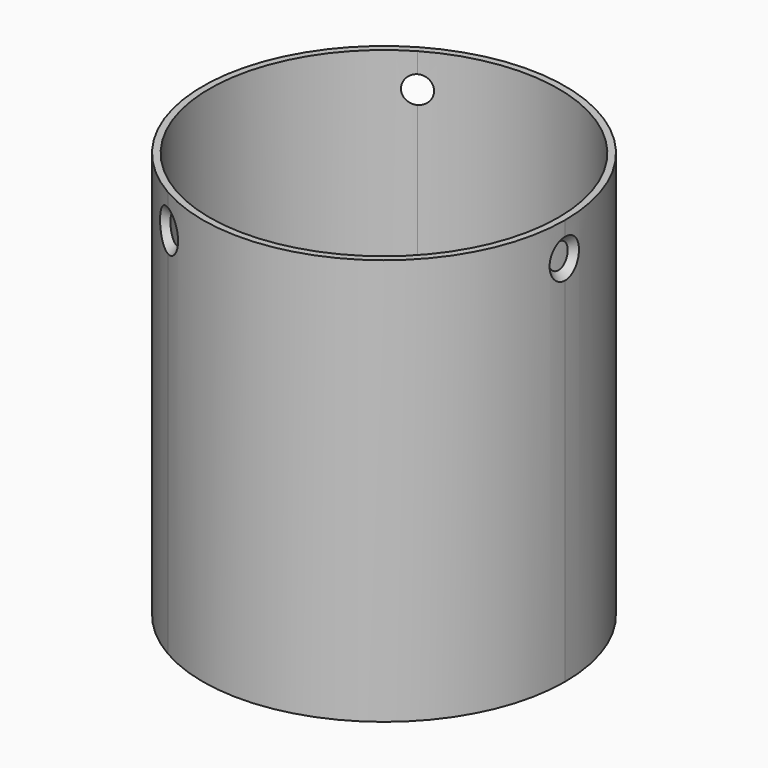
from build123d import *

# Parameters (mm, degrees)
F1_DEPTH             = 60
F2_DEPTH             = 58
F9_D                 = 3.2
F9_DEPTH             = 4
F9_CSINK_D           = 6
F9_CSINK_ANGLE       = 90
F9_TIP               = 0.9613769904
F9_ON_F6_D           = 3.2
F9_ON_F6_DEPTH       = 4
F9_ON_F6_CSINK_D     = 6
F9_ON_F6_CSINK_ANGLE = 90
F9_ON_F6_TIP         = 0.9613769904
F9_ON_F8_D           = 3.2
F9_ON_F8_DEPTH       = 4
F9_ON_F8_CSINK_D     = 6
F9_ON_F8_CSINK_ANGLE = 90
F9_ON_F8_TIP         = 0.9613769904


# Not quite as in the source:
# - a feature names something its author has since deleted; it is built from what else it names


with BuildPart() as f1:
    # F0 (on Top) → F1 (new body)
    with BuildSketch(Plane.XY):
        with BuildLine():
            ThreePointArc((-13.375, -23.1661795512), (13.375, -23.1661795512), (26.75, 0))
            ThreePointArc((26.75, 0), (13.375, 23.1661795512), (-13.375, 23.1661795512))
            Line((-13.375, 23.1661795512), (-12.875, 22.3001541474))
            ThreePointArc((-12.875, 22.3001541474), (12.875, 22.3001541474), (25.75, 0))
            ThreePointArc((25.75, 0), (12.875, -22.3001541474), (-12.875, -22.3001541474))
            Line((-12.875, -22.3001541474), (-13.375, -23.1661795512))
        make_face()
        with BuildLine():
            Line((-12.875, 22.3001541474), (-13.375, 23.1661795512))
            ThreePointArc((-13.375, 23.1661795512), (-26.75, 0), (-13.375, -23.1661795512))
            Line((-13.375, -23.1661795512), (-12.875, -22.3001541474))
            ThreePointArc((-12.875, -22.3001541474), (-25.75, 0), (-12.875, 22.3001541474))
        make_face()
        with BuildLine():
            ThreePointArc((25.75, 0), (12.875, 22.3001541474), (-12.875, 22.3001541474))
            Line((-12.875, 22.3001541474), (0, 0))
            Line((0, 0), (-12.875, -22.3001541474))
            ThreePointArc((-12.875, -22.3001541474), (12.875, -22.3001541474), (25.75, 0))
        make_face()
        with BuildLine():
            Line((0, 0), (-12.875, 22.3001541474))
            ThreePointArc((-12.875, 22.3001541474), (-25.75, 0), (-12.875, -22.3001541474))
            Line((-12.875, -22.3001541474), (0, 0))
        make_face()
    extrude(amount=-F1_DEPTH)

    # F0 (on Top) → F2 (cut)
    with BuildSketch(Plane.XY):
        with BuildLine():
            ThreePointArc((25.75, 0), (12.875, 22.3001541474), (-12.875, 22.3001541474))
            Line((-12.875, 22.3001541474), (0, 0))
            Line((0, 0), (-12.875, -22.3001541474))
            ThreePointArc((-12.875, -22.3001541474), (12.875, -22.3001541474), (25.75, 0))
        make_face()
        with BuildLine():
            Line((0, 0), (-12.875, 22.3001541474))
            ThreePointArc((-12.875, 22.3001541474), (-25.75, 0), (-12.875, -22.3001541474))
            Line((-12.875, -22.3001541474), (0, 0))
        make_face()
    extrude(amount=-F2_DEPTH, mode=Mode.SUBTRACT)

    # F9
    with Locations(Plane(origin=(-13.375, 23.1661795512, 0), x_dir=(-0.8660254038, -0.5, 0), z_dir=(-0.5, 0.8660254038, 0))):
        with Locations((0, -5)):
            CounterSinkHole(F9_D / 2, F9_CSINK_D / 2, depth=F9_DEPTH, counter_sink_angle=F9_CSINK_ANGLE)
            with Locations((0, 0, -(F9_DEPTH + F9_TIP / 2))):  # 118° drill point
                Cone(0, F9_D / 2, F9_TIP, mode=Mode.SUBTRACT)

    # F9 on F6
    with Locations(Plane.YZ.offset(26.9)):
        with Locations((0, -5)):
            CounterSinkHole(F9_ON_F6_D / 2, F9_ON_F6_CSINK_D / 2, depth=F9_ON_F6_DEPTH, counter_sink_angle=F9_ON_F6_CSINK_ANGLE)
            with Locations((0, 0, -(F9_ON_F6_DEPTH + F9_ON_F6_TIP / 2))):  # 118° drill point
                Cone(0, F9_ON_F6_D / 2, F9_ON_F6_TIP, mode=Mode.SUBTRACT)

    # F9 on F8
    with Locations(Plane(origin=(-13.375, -23.1661795512, 0), x_dir=(0.8660254038, -0.5, 0), z_dir=(-0.5, -0.8660254038, 0))):
        with Locations((0, -5)):
            CounterSinkHole(F9_ON_F8_D / 2, F9_ON_F8_CSINK_D / 2, depth=F9_ON_F8_DEPTH, counter_sink_angle=F9_ON_F8_CSINK_ANGLE)
            with Locations((0, 0, -(F9_ON_F8_DEPTH + F9_ON_F8_TIP / 2))):  # 118° drill point
                Cone(0, F9_ON_F8_D / 2, F9_ON_F8_TIP, mode=Mode.SUBTRACT)


solid = f1.part
